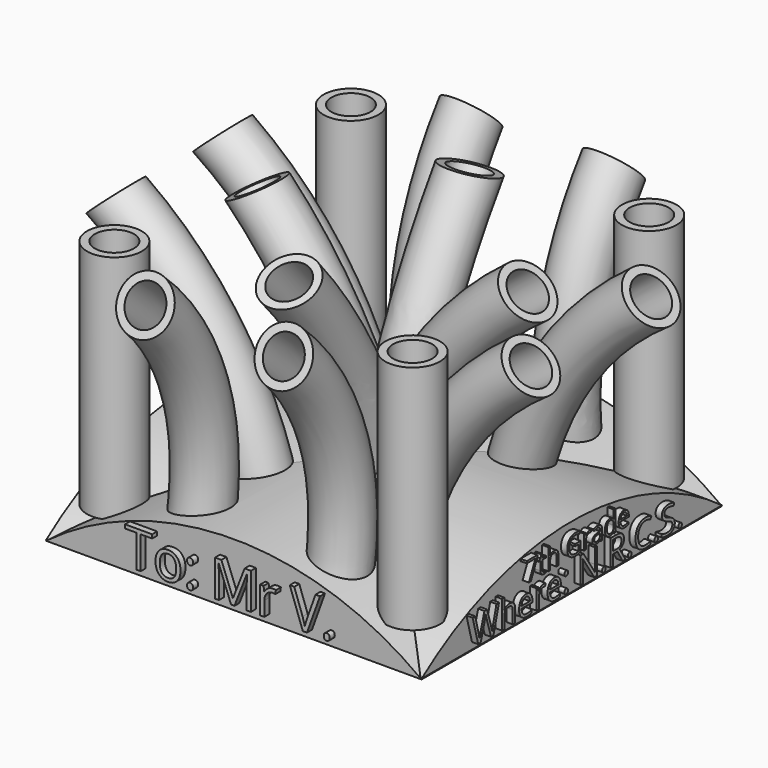
from build123d import *

# Parameters (mm, degrees)
F1_DEPTH      = 76.2
F1_DEPTH_BACK = 76.2
F3_DEPTH      = 76.2
F3_DEPTH_BACK = 76.2
F4_R          = 11.1125
F4_R_2        = 7.9375
F13_R         = 11.1125
F13_R_2       = 7.9375
F16_R         = 11.1125
F16_R_2       = 7.9375
F16_R_3       = 8.0589675726
F19_R         = 11.1125
F19_R_2       = 7.9375
F22_R         = 11.1125
F22_R_2       = 7.9375
F25_TEXT_SIZE = 20.6083318511
F26_DEPTH     = 2.54
F27_TEXT_SIZE = 16.2324850017
F28_DEPTH     = 2.54
F29_R         = 11.1125
F29_R_2       = 7.9375
F32_TEXT_SIZE = 13.9239137238
F33_DEPTH     = 2.54
F34_TEXT_SIZE = 14.8962840969
F35_DEPTH     = 2.54
F36_TEXT_SIZE = 11.3354422775
F37_DEPTH     = 2.54


# Not quite as in the source:
# - Text() gives the source's letters only with a copy of the font that has no kerning and outlines rounded to 1/6400 em; it was checked with that copy


with BuildPart() as f1:
    # F0 (on Front) → F1 (new body, two sides)
    with BuildSketch(Plane.XZ) as f1_sk:
        with BuildLine():
            Line((-76.2, -11.5132788196), (0, -11.5132788196))
            Line((0, -11.5132788196), (76.2, -11.5132788196))
            ThreePointArc((76.2, -11.5132788196), (0, 13.8867211804), (-76.2, -11.5132788196))
        make_face()
    extrude(amount=F1_DEPTH)
    extrude(f1_sk.sketch, amount=-F1_DEPTH_BACK)

    # F2 (on Right) → F3 (join, two sides)
    with BuildSketch(Plane.YZ) as f3_sk:
        with BuildLine():
            Line((-76.2, -11.2218027934), (0, -11.2218027934))
            Line((0, -11.2218027934), (76.2, -11.2218027934))
            ThreePointArc((76.2, -11.2218027934), (0, 14.0613699332), (-76.2, -11.2218027934))
        make_face()
    extrude(amount=F3_DEPTH)
    extrude(f3_sk.sketch, amount=-F3_DEPTH_BACK)

    # F6: sweep along a path in F5
    with BuildLine(Plane.XZ) as f6_path:
        ThreePointArc((0, 0), (-19.5522068788, 49.5167473265), (-51.3727739453, 92.197522521))
    # F4 (on Top) → F6 (sweep)
    with BuildSketch(Plane.XY):
        Circle(F4_R)
        Circle(F4_R_2, mode=Mode.SUBTRACT)
    sweep(path=f6_path.line)

    # F8: sweep along a path in F7
    with BuildLine(Plane.XZ) as f8_path:
        ThreePointArc((58.3417899907, 90.3114303946), (20.6692757694, 50.64781826), (0, 0))
    # F4 (on Top) → F8 (sweep)
    with BuildSketch(Plane.XY):
        Circle(F4_R)
        Circle(F4_R_2, mode=Mode.SUBTRACT)
    sweep(path=f8_path.line)

    # F10: sweep along a path in F9
    with BuildLine(Plane.YZ) as f10_path:
        ThreePointArc((1.2653707527, 0), (-16.9144069977, 50.5201720787), (-47.0074340701, 94.98590976))
    # F4 (on Top) → F10 (sweep)
    with BuildSketch(Plane.XY):
        Circle(F4_R)
        Circle(F4_R_2, mode=Mode.SUBTRACT)
    sweep(path=f10_path.line)

    # F12: sweep along a path in F11
    with BuildLine(Plane.YZ) as f12_path:
        ThreePointArc((43.4447899461, 97.6759791374), (17.3642099756, 50.776443971), (0, 0))
    # F4 (on Top) → F12 (sweep)
    with BuildSketch(Plane.XY):
        Circle(F4_R)
        Circle(F4_R_2, mode=Mode.SUBTRACT)
    sweep(path=f12_path.line)

    # F15: sweep along a path in F14
    with BuildLine(Plane.XZ) as f15_path:
        ThreePointArc((-26.3838544488, 0), (-48.4910818159, 49.921825934), (-87.1532261372, 88.4725302458))
    # F13 (on Top) → F15 (sweep)
    with BuildSketch(Plane.XY):
        with Locations((-26.3300575316, 27.1644610912)):
            Circle(F13_R)
        with Locations((-26.3300575316, 27.1644610912)):
            Circle(F13_R_2, mode=Mode.SUBTRACT)
        with Locations((-26.3300575316, -26.9790366292)):
            Circle(F13_R)
        with Locations((-26.3300575316, -26.9790366292)):
            Circle(F13_R_2, mode=Mode.SUBTRACT)
    sweep(path=f15_path.line)

    # F18: sweep along a path in F17
    with BuildLine(Plane.XZ) as f18_path:
        ThreePointArc((84.5166519284, 84.7960859537), (48.8514215664, 47.7588500152), (29.8025961965, 0))
    # F16 (on Top) → F18 (sweep)
    with BuildSketch(Plane.XY):
        with Locations((29.7527406365, 29.9458056688)):
            Circle(F16_R)
        with Locations((29.7527406365, 29.9458056688)):
            Circle(F16_R_2, mode=Mode.SUBTRACT)
        with Locations((29.7527406365, -31.0583431274)):
            Circle(F16_R)
        with Locations((29.7527406365, -31.0583431274)):
            Circle(F16_R_3, mode=Mode.SUBTRACT)
    sweep(path=f18_path.line)

    # F21: sweep along a path in F20
    with BuildLine(Plane.YZ) as f21_path:
        ThreePointArc((-61.0909163952, 0), (-61.755128114, 50.4476824758), (-87.9446342587, 93.56983006))
    # F19 (on Top) → F21 (sweep)
    with BuildSketch(Plane.XY):
        with Locations((-26.4752153307, -61.0968619585)):
            Circle(F19_R)
        with Locations((-26.4752153307, -61.0968619585)):
            Circle(F19_R_2, mode=Mode.SUBTRACT)
        with Locations((29.7079402953, -61.0968619585)):
            Circle(F19_R)
        with Locations((29.7079402953, -61.0968619585)):
            Circle(F19_R_2, mode=Mode.SUBTRACT)
    sweep(path=f21_path.line)

    # F24: sweep along a path in F23
    with BuildLine(Plane.YZ) as f24_path:
        ThreePointArc((81.9397494197, 92.5211086869), (61.1694843513, 48.5638676713), (58.8905140758, 0))
    # F22 (on Top) → F24 (sweep)
    with BuildSketch(Plane.XY):
        with Locations((-30.2562434226, 58.9883513749)):
            Circle(F22_R)
        with Locations((-30.2562434226, 58.9883513749)):
            Circle(F22_R_2, mode=Mode.SUBTRACT)
        with Locations((27.6901517063, 58.9883513749)):
            Circle(F22_R)
        with Locations((27.6901517063, 58.9883513749)):
            Circle(F22_R_2, mode=Mode.SUBTRACT)
    sweep(path=f24_path.line)

    # F25 (on face) → F26 (join)
    with BuildSketch(Plane.XZ.offset(76.2)):
        with Locations((-42.3098713059, -8.206236978)):
            Text('To: Mr V.', F25_TEXT_SIZE, font='Open Sans', text_align=(TextAlign.LEFT, TextAlign.BOTTOM))
    extrude(amount=F26_DEPTH)

    # F27 (on face) → F28 (join)
    with BuildSketch(Plane(origin=(0, 76.2, 0), x_dir=(-1, 0, 0), z_dir=(0, 1, 0))):
        with Locations((-48.6103765697, -7.4719362892)):
            Text('From: Karter', F27_TEXT_SIZE, font='Open Sans', text_align=(TextAlign.LEFT, TextAlign.BOTTOM))
    extrude(amount=F28_DEPTH)

    # F31: sweep along a path in F30
    with BuildLine(Plane.XZ) as f31_path:
        Line((-61.4389404655, 0), (-61.4389404655, 93.8769355416))
    # F29 (on Top) → F31 (sweep)
    with BuildSketch(Plane.XY):
        with Locations((-61.2838976085, 59.8267093301)):
            Circle(F29_R)
        with Locations((-61.2838976085, 59.8267093301)):
            Circle(F29_R_2, mode=Mode.SUBTRACT)
        with Locations((59.7812645137, 59.8267093301)):
            Circle(F29_R)
        with Locations((59.7812645137, 59.8267093301)):
            Circle(F29_R_2, mode=Mode.SUBTRACT)
        with Locations((59.7812645137, -60.2007545531)):
            Circle(F29_R)
        with Locations((59.7812645137, -60.2007545531)):
            Circle(F29_R_2, mode=Mode.SUBTRACT)
        with Locations((-61.2838976085, -60.2007545531)):
            Circle(F29_R)
        with Locations((-61.2838976085, -60.2007545531)):
            Circle(F29_R_2, mode=Mode.SUBTRACT)
    sweep(path=f31_path.line)

    # F32 (on face) → F33 (join)
    with BuildSketch(Plane(origin=(-76.2, 0, 0), x_dir=(0, -1, 0), z_dir=(-1, 0, 0))):
        with Locations((-56.7388606188, -9.2879079299)):
            Text('When: 2016-2017', F32_TEXT_SIZE, font='Open Sans', text_align=(TextAlign.LEFT, TextAlign.BOTTOM))
    extrude(amount=F33_DEPTH)

    # F34 (on face) → F35 (join)
    with BuildSketch(Plane.YZ.offset(76.2)):
        with Locations((-53.6475706482, -8.5029342644)):
            Text('Where: N.R.C.S.', F34_TEXT_SIZE, font='Open Sans', text_align=(TextAlign.LEFT, TextAlign.BOTTOM))
    extrude(amount=F35_DEPTH)

    # F36 (on face) → F37 (join)
    with BuildSketch(Plane.YZ.offset(76.2)):
        with Locations((-26.5081088823, 3.1131286602)):
            Text('7th Grade', F36_TEXT_SIZE, font='Open Sans', text_align=(TextAlign.LEFT, TextAlign.BOTTOM))
    extrude(amount=F37_DEPTH)


solid = f1.part
